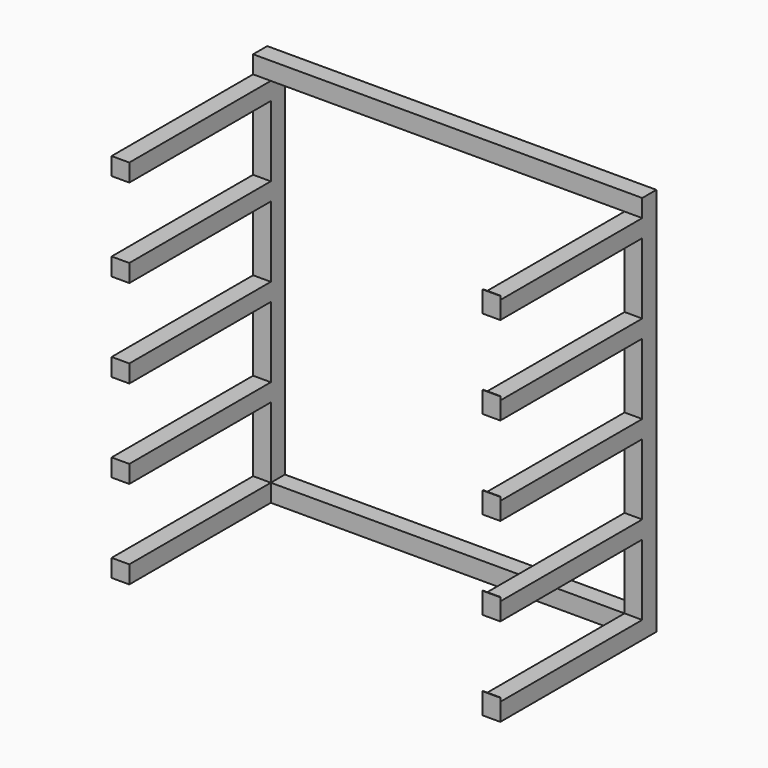
from build123d import *

# Parameters (mm, degrees)
F0_W     = 2000
F0_H     = 100
F1_DEPTH = 100
F2_W     = 100
F2_H     = 100
F3_DEPTH = 1000
F5_DEPTH = 100


# Not quite as in the source:
# - the program builds the solid bodies; features that only make, move or delete a surface that nothing else refers to are left out


with BuildPart() as f1:
    # F0 (on Front) → F1 (new body)
    with BuildSketch(Plane.XZ):
        Polygon((100, 0), (0, 0), (0, -2200), (100, -2200), (100, -2100), (100, -100), align=None)
        with Locations((1100, -2150)):
            Rectangle(F0_W, F0_H)
        Polygon((2200, 0), (2100, 0), (2100, -100), (2100, -2100), (2100, -2200), (2200, -2200), align=None)
        with Locations((1100, -50)):
            Rectangle(F0_W, F0_H)
    extrude(amount=F1_DEPTH)

    # F2 (on face) → F3 (join)
    with BuildSketch(Plane.XZ.offset(100)):
        with Locations((50, -150)):
            Rectangle(F2_W, F2_H)
        with Locations((50, -650)):
            Rectangle(F2_W, F2_H)
        with Locations((50, -1150)):
            Rectangle(F2_W, F2_H)
        with Locations((50, -1650)):
            Rectangle(F2_W, F2_H)
        with Locations((50, -2150)):
            Rectangle(F2_W, F2_H)
        with Locations((2150, -2150)):
            Rectangle(F2_W, F2_H)
        with Locations((2150, -1650)):
            Rectangle(F2_W, F2_H)
        with Locations((2150, -1150)):
            Rectangle(F2_W, F2_H)
        with Locations((2150, -650)):
            Rectangle(F2_W, F2_H)
        with Locations((2150, -150)):
            Rectangle(F2_W, F2_H)
    extrude(amount=F3_DEPTH)


with BuildPart() as f5:
    # F4 (on face) → F5 (new body)
    with BuildSketch(Plane.YZ.offset(2200)):
        Polygon((-1103, -2200), (-1100, -2200), (-1100, -2100), (-1100, -2080), (-1103, -2080), align=None)
    extrude(amount=-F5_DEPTH)


with BuildPart() as f5b:
    # F4 (on face) → F5, piece 2 (new body)
    with BuildSketch(Plane.YZ.offset(2200)):
        Polygon((-1103, -1700), (-1100, -1700), (-1100, -1600), (-1100, -1580), (-1103, -1580), align=None)
    extrude(amount=-F5_DEPTH)


with BuildPart() as f5c:
    # F4 (on face) → F5, piece 3 (new body)
    with BuildSketch(Plane.YZ.offset(2200)):
        Polygon((-1100, -1200), (-1100, -1100), (-1100, -1080), (-1103, -1080), (-1103, -1200), align=None)
    extrude(amount=-F5_DEPTH)


with BuildPart() as f5d:
    # F4 (on face) → F5, piece 4 (new body)
    with BuildSketch(Plane.YZ.offset(2200)):
        Polygon((-1100, -700), (-1100, -600), (-1100, -580), (-1103, -580), (-1103, -700), align=None)
    extrude(amount=-F5_DEPTH)


with BuildPart() as f5e:
    # F4 (on face) → F5, piece 5 (new body)
    with BuildSketch(Plane.YZ.offset(2200)):
        Polygon((-1103, -200), (-1100, -200), (-1100, -100), (-1100, -80), (-1103, -80), align=None)
    extrude(amount=-F5_DEPTH)


solid = Compound([f1.part, f5.part, f5b.part, f5c.part, f5d.part, f5e.part])
